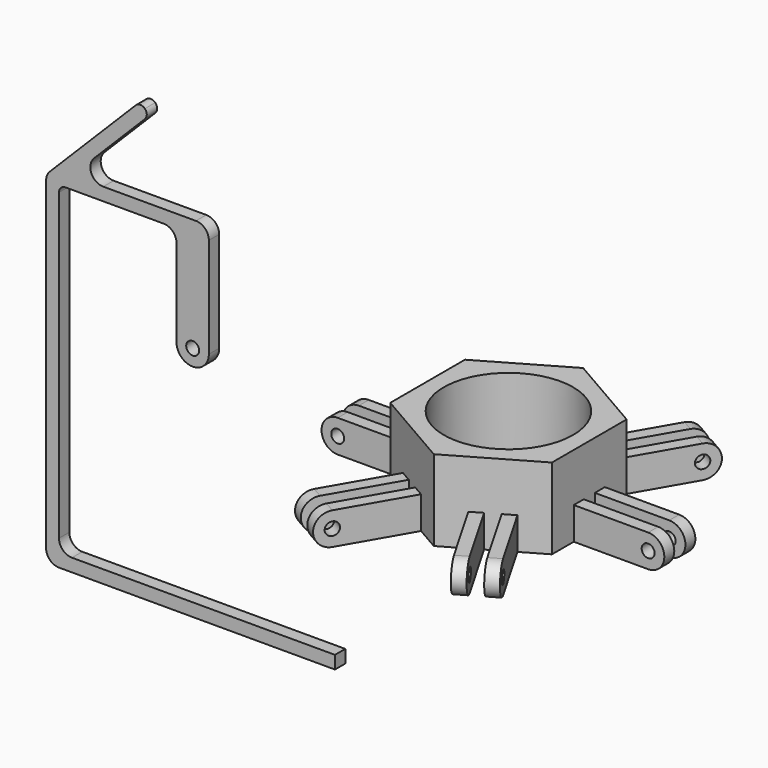
from build123d import *

# Parameters (mm, degrees)
F0_R     = 2
F1_DEPTH = 4
F2_R     = 2
F3_DEPTH = 6
F4_W     = 23
F4_H     = 2.15
F5_DEPTH = 10
F7_R     = 20
F8_DEPTH = 25
F9_COUNT = 6


with BuildPart() as f1:
    # F0 (on Front) → F1 (new body)
    with BuildSketch(Plane.XZ):
        with BuildLine():
            Line((-139.7852453673, 43.9352564364), (-139.7852453673, -56.1412286615))
            ThreePointArc((-139.7852453673, -56.1412286615), (-138.6136724921, -58.9696557863), (-135.7852453673, -60.1412286615))
            Line((-135.7852453673, -60.1412286615), (-50.451497823, -60.1412286615))
            Line((-50.451497823, -60.1412286615), (-50.451497823, -56.1412286615))
            Line((-50.451497823, -56.1412286615), (-131.7852453673, -56.1412286615))
            ThreePointArc((-131.7852453673, -56.1412286615), (-134.6136724921, -54.9696557863), (-135.7852453673, -52.1412286615))
            Line((-135.7852453673, -52.1412286615), (-135.7852453673, 42.0244794162))
            ThreePointArc((-135.7852453673, 42.0244794162), (-135.1994589297, 43.4386929786), (-133.7852453673, 44.0244794162))
            Line((-133.7852453673, 44.0244794162), (-103.451497823, 44.0244794162))
            ThreePointArc((-103.451497823, 44.0244794162), (-100.6230706983, 42.8529065409), (-99.451497823, 40.0244794162))
            Line((-99.451497823, 40.0244794162), (-99.451497823, 13.0244794162))
            ThreePointArc((-99.451497823, 13.0244794162), (-97.9870317289, 9.4889455103), (-94.451497823, 8.0244794162))
            ThreePointArc((-94.451497823, 8.0244794162), (-90.9159639171, 9.4889455103), (-89.451497823, 13.0244794162))
            Line((-89.451497823, 13.0244794162), (-89.451497823, 44.0244794162))
            ThreePointArc((-89.451497823, 44.0244794162), (-90.6230706983, 46.8529065409), (-93.451497823, 48.0244794162))
            Line((-93.451497823, 48.0244794162), (-122.0909434094, 48.0244794162))
            ThreePointArc((-122.0909434094, 48.0244794162), (-125.7846392397, 50.4893536517), (-124.9260872271, 54.8461738597))
            Line((-124.9260872271, 54.8461738597), (-109.2275817345, 70.6195049861))
            ThreePointArc((-109.2275817345, 70.6195049861), (-108.6451592961, 72.0351072797), (-109.2343064216, 73.4479241167))
            ThreePointArc((-109.2343064216, 73.4479241167), (-110.6499087152, 74.0303465551), (-112.0627255523, 73.4411994296))
            Line((-112.0627255523, 73.4411994296), (-138.6203891851, 46.75695088))
            ThreePointArc((-138.6203891851, 46.75695088), (-139.4825805747, 45.4615959676), (-139.7852453673, 43.9352564364))
        make_face()
        with Locations((-94.451497823, 13.0244794162)):
            Circle(F0_R, mode=Mode.SUBTRACT)
    extrude(amount=F1_DEPTH)


with BuildPart() as f3:
    # F2 (on Front) → F3 (new body, symmetric)
    with BuildSketch(Plane.XZ):
        with BuildLine():
            Line((-25, 10), (-48, 10))
            ThreePointArc((-48, 10), (-51.5355339059, 8.5355339059), (-53, 5))
            ThreePointArc((-53, 5), (-51.5355339059, 1.4644660941), (-48, 0))
            Line((-48, 0), (-25, 0))
            Line((-25, 0), (-25, 10))
        make_face()
        with Locations((-48, 5)):
            Circle(F2_R, mode=Mode.SUBTRACT)
    extrude(amount=F3_DEPTH, both=True)

    # F4 (on face) → F5 (cut, through all)
    with BuildSketch(Plane.XY.offset(10)):
        with Locations((-36.5, 1.075)):
            Rectangle(F4_W, F4_H)
        Polygon((-48, 2.15), (-53, 2.15), (-53, -2.15), (-25, -2.15), (-25, 0), (-48, 0), align=None)
    extrude(amount=-F5_DEPTH, mode=Mode.SUBTRACT)


with BuildPart() as f8:
    # F7 (on face) → F8 (new body)
    with BuildSketch(Plane.XY):
        Polygon((0, 28.8675134595), (-25, 14.4337567297), (-25, -14.4337567297), (0, -28.8675134595), (25, -14.4337567297), (25, 14.4337567297), align=None)
        Circle(F7_R, mode=Mode.SUBTRACT)
    extrude(amount=F8_DEPTH)


with BuildPart() as f9_1:
    # F9: instance of F3
    add(f3.part.rotate(Axis((0, 0, 12.9298158377), (0, 0, 1)), 1 * 360 / F9_COUNT))


with BuildPart() as f9_2:
    # F9: instance of F3
    add(f3.part.rotate(Axis((0, 0, 12.9298158377), (0, 0, 1)), 2 * 360 / F9_COUNT))


with BuildPart() as f9_3:
    # F9: instance of F3
    add(f3.part.rotate(Axis((0, 0, 12.9298158377), (0, 0, 1)), 3 * 360 / F9_COUNT))


with BuildPart() as f9_4:
    # F9: instance of F3
    add(f3.part.rotate(Axis((0, 0, 12.9298158377), (0, 0, 1)), 4 * 360 / F9_COUNT))


with BuildPart() as f9_5:
    # F9: instance of F3
    add(f3.part.rotate(Axis((0, 0, 12.9298158377), (0, 0, 1)), 5 * 360 / F9_COUNT))


solid = Compound([f1.part, f3.part, f8.part, f9_1.part, f9_2.part, f9_3.part, f9_4.part, f9_5.part])
